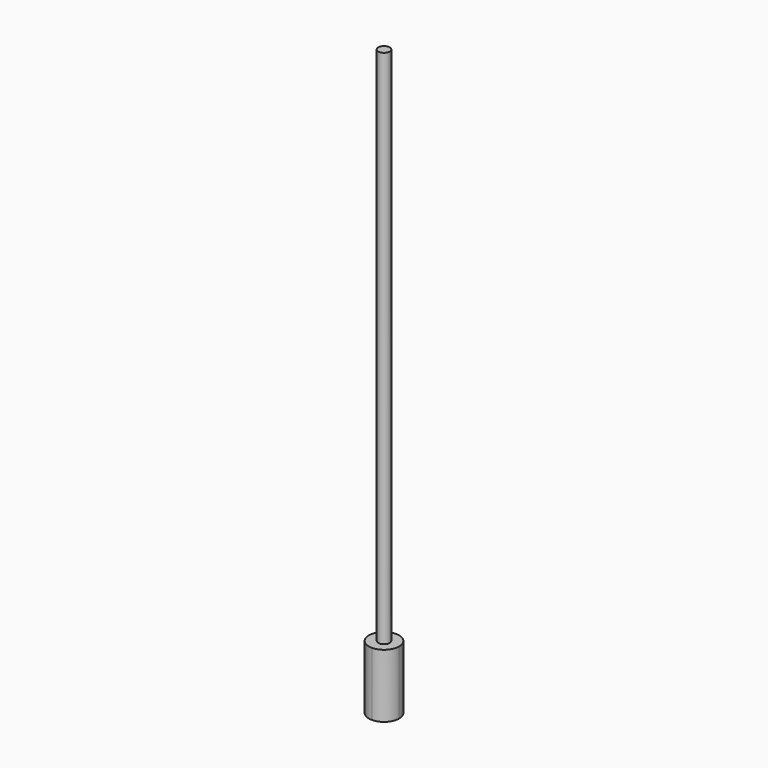
from build123d import *

# Parameters (mm, degrees)
F0_W        = 11.43
F0_H        = 11.43
F0_R        = 2.15265
F1_DEPTH    = 22.4125
F2_W        = 11.43
F2_H        = 11.43
F3_DEPTH    = 1.5875
F4_R        = 1.35255
F5_REACH    = 15.2565891076
F6_T1_DEPTH = 52.575
F7_R        = 2.15265
F8_DEPTH    = 196.85


# Not quite as in the source:
# - a fillet or chamfer that OpenCascade refuses, or shapes differently, is made with other operations: its cross-section is extruded or revolved along the edge and cut away or added


with BuildPart() as f1:
    # F0 (on Top) → F1 (new body)
    with BuildSketch(Plane.XY):
        Rectangle(F0_W, F0_H)
        Circle(F0_R, mode=Mode.SUBTRACT)
    extrude(amount=F1_DEPTH)

    # F2 (on face) → F3 (join)
    with BuildSketch(Plane.XY.offset(22.4125)):
        Rectangle(F2_W, F2_H)
    extrude(amount=F3_DEPTH)

    f5_end = f1.faces().sort_by_distance((-2.15265, 0, 11.20625))[0]
    # F4 (on face) → F5 (cut, up to a face of the model that its end follows)
    with BuildSketch(Plane(origin=(-5.715, 0, 0), x_dir=(0, -1, 0), z_dir=(-1, 0, 0))):
        with Locations((0, 11.20625)):
            Circle(F4_R)
    f5_long = extrude(amount=-F5_REACH, mode=Mode.PRIVATE)
    add(split(f5_long, bisect_by=f5_end, keep=Keep.ALL, mode=Mode.PRIVATE).solids().sort_by_distance((-5.715, 0, 11.20625))[0], mode=Mode.SUBTRACT)

    # F6: fillet of radius 5.715 on 4 edges, made by hand

    # F6_s2 → F6_t1 (cut)
    with BuildSketch(Plane.XY.offset(-14.2875)):
        with BuildLine():
            ThreePointArc((0, -5.715), (-4.0411152545, -4.0411152545), (-5.715, 0))
            Line((-5.715, 0), (-5.715, -5.715))
            Line((-5.715, -5.715), (0, -5.715))
        make_face()
        with BuildLine():
            ThreePointArc((0, -5.715), (4.0411152545, -4.0411152545), (5.715, 0))
            Line((5.715, 0), (5.715, -5.715))
            Line((5.715, -5.715), (0, -5.715))
        make_face()
        with BuildLine():
            ThreePointArc((-5.715, 0), (-4.0411152545, 4.0411152545), (0, 5.715))
            Line((0, 5.715), (-5.715, 5.715))
            Line((-5.715, 5.715), (-5.715, 0))
        make_face()
        with BuildLine():
            ThreePointArc((5.715, 0), (4.0411152545, 4.0411152545), (0, 5.715))
            Line((0, 5.715), (5.715, 5.715))
            Line((5.715, 5.715), (5.715, 0))
        make_face()
    extrude(amount=F6_T1_DEPTH, mode=Mode.SUBTRACT)

    # F7 (on face) → F8 (join)
    with BuildSketch(Plane.XY.offset(24)):
        Circle(F7_R)
    extrude(amount=F8_DEPTH)


solid = f1.part
